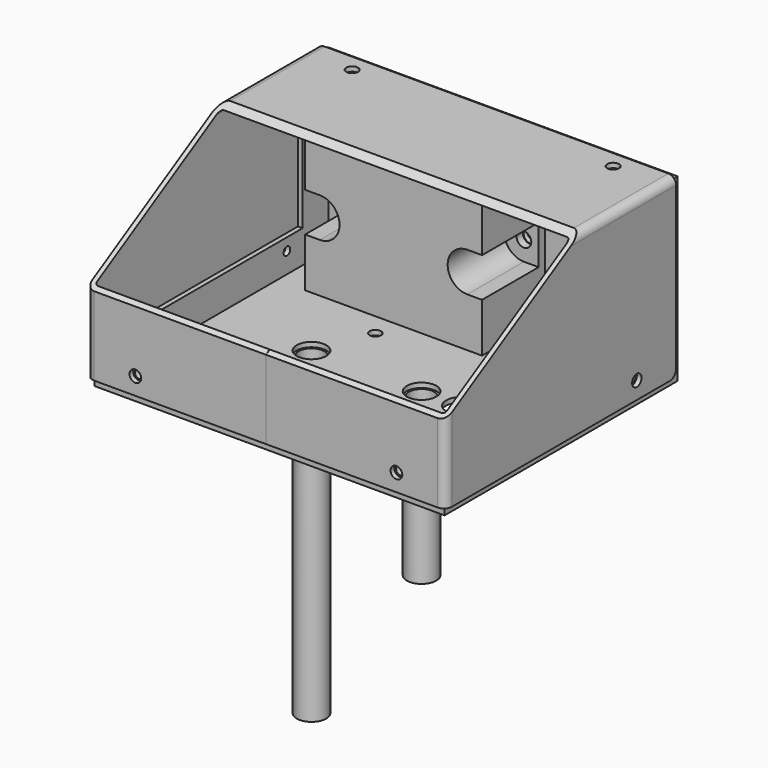
from build123d import *

# Parameters (mm, degrees)
F1_DEPTH         = 116.078
F2_R             = 2.54
F3_T             = -1.524
F5_DEPTH         = 113.03
F6_T             = -1.524
F7_W             = 57.15
F7_H             = 44.45
F8_DEPTH         = 25.4
F10_DEPTH        = 22.86
F11_R            = 2.3749
F12_DEPTH        = 26.925
F13_R            = 4.7625
F14_DEPTH        = 1.524
F15_R            = 4.7625
F15_R_2          = 4.1275
F16_DEPTH        = 50.8
F17_DEPTH        = 101.6
F18_R            = 1.8288
F19_DEPTH        = 59.691
F20_R            = 2.15265
F21_DEPTH        = 1.525
F22_R            = 9.525
F23_DEPTH        = 1.525
F27_D            = 3.7973
F27_ON_F25_D     = 3.7973
F27_ON_F24_D     = 3.7973
F28_D            = 2.7051
F29_D            = 2.7051
F29_DEPTH        = 12.7
F29_START        = 1.524
F29_TIP          = 0.8126940303
F29_ON_F25_D     = 2.7051
F29_ON_F25_DEPTH = 12.7
F29_ON_F25_START = 1.524
F29_ON_F25_TIP   = 0.8126940303
F30_W            = 0.0254
F30_H            = 69.686152041
F31_DEPTH        = 25.4
F32_R            = 2.54


with BuildPart() as f1:
    # F0 (on Right) → F1 (new body)
    with BuildSketch(Plane.YZ):
        Polygon((0, 25.4), (0, 0), (93.0926131403, 0), (93.0926131403, 57.15), (54.9926131403, 57.15), align=None)
    extrude(amount=F1_DEPTH)

    # F2
    f2_edges = [f1.edges().sort_by_distance(p)[0] for p in [
        (116.078, 74.042613, 57.15),
        (116.078, 0, 12.7),
        (0, 0, 12.7),
        (0, 74.042613, 57.15),
    ]]
    fillet(f2_edges, radius=F2_R)

    # F3
    f3_openings = [f1.faces().sort_by_distance(p)[0] for p in [
        (58.039, 93.092613, 28.563304),
        (58.039, 46.558092, 0),
        (58.039, 27.488057, 41.270237),
    ]]
    offset(amount=F3_T, openings=f3_openings)

    # F27 (through all)
    with Locations(Plane.XY.offset(57.15)):
        with Locations((100.203, 87.5046131403), (15.875, 87.5046131403)):
            Hole(F27_D / 2)

    # F27 on F25 (through all)
    with Locations(Plane.XZ):
        with Locations((15.875, 5.588), (100.203, 5.588)):
            Hole(F27_ON_F25_D / 2)

    # F27 on F24 (through all)
    with Locations(Plane(origin=(0, 0, 0), x_dir=(0, -1, 0), z_dir=(-1, 0, 0))):
        with Locations((-77.2176131403, 5.588)):
            Hole(F27_ON_F24_D / 2)

    # F30 (on face) → F31 (cut)
    with BuildSketch(Plane.XZ):
        with Locations((58.0517, 34.8430760205)):
            Rectangle(F30_W, F30_H)
    extrude(amount=-F31_DEPTH, mode=Mode.SUBTRACT)

    # F32
    f32_edges = [f1.edges().sort_by_distance(p)[0] for p in [
        (0.762, 93.092613, 0),
        (115.316, 93.092613, 0),
    ]]
    fillet(f32_edges, radius=F32_R)


with BuildPart() as f5:
    # F4 (on face) → F5 (new body, through all)
    with BuildSketch(Plane(origin=(114.554, 0, 0), x_dir=(0, -1, 0), z_dir=(-1, 0, 0))):
        Polygon((-1.524, 9.525), (-83.5676131403, 9.525), (-83.5676131403, 55.626), (-93.0926131403, 55.626), (-95.6326131403, 55.626), (-95.6326131403, -2.54), (-1.524, -2.54), (-1.524, 0), align=None)
    extrude(amount=F5_DEPTH)

    # F6
    f6_openings = [f5.faces().sort_by_distance(p)[0] for p in [
        (58.039, 83.567613, 32.5755),
        (58.039, 42.545807, 9.525),
    ]]
    offset(amount=F6_T, openings=f6_openings)

    # F13 (on face) → F14 (cut, through all)
    with BuildSketch(Plane(origin=(0, 0, -2.54), x_dir=(1, 0, 0), z_dir=(0, 0, -1))):
        with Locations((82.169, -48.5783125154)):
            Circle(F13_R)
        with Locations((69.469, -48.5783125154)):
            Circle(F13_R)
        with Locations((33.909, -48.5783125154)):
            Circle(F13_R)
    extrude(amount=-F14_DEPTH, mode=Mode.SUBTRACT)

    # F18 (on face) → F19 (cut, through all)
    with BuildSketch(Plane(origin=(0, 0, -2.54), x_dir=(1, 0, 0), z_dir=(0, 0, -1))):
        with Locations((40.5765, -31.1158125154)):
            Circle(F18_R)
        with Locations((75.5015, -31.1158125154)):
            Circle(F18_R)
        with Locations((75.5015, -66.0408125154)):
            Circle(F18_R)
        with Locations((40.5765, -66.0408125154)):
            Circle(F18_R)
    extrude(amount=-F19_DEPTH, mode=Mode.SUBTRACT)

    # F20 (on face) → F21 (cut, through all)
    with BuildSketch(Plane.XZ.offset(-94.1086131403)):
        with Locations((20.5105, 24.257)):
            Circle(F20_R)
        with Locations((68.1355, 24.257)):
            Circle(F20_R)
    extrude(amount=-F21_DEPTH, mode=Mode.SUBTRACT)

    # F22 (on face) → F23 (cut, through all)
    with BuildSketch(Plane.XZ.offset(-94.1086131403)):
        with Locations((92.964, 19.05)):
            Circle(F22_R)
    extrude(amount=-F23_DEPTH, mode=Mode.SUBTRACT)

    # F28 (through all)
    with Locations(Plane(origin=(0, 0, 0), x_dir=(0, -1, 0), z_dir=(-1, 0, 0))):
        with Locations((-77.2176131403, 5.588)):
            Hole(F28_D / 2)

    # F29
    # its depths count from where the whole tool has entered the part; down to there all is cleared
    with Locations(Plane.XY.offset(57.15).offset(-F29_START)):
        with Locations((15.875, 87.5046131403), (100.203, 87.5046131403)):
            Hole(F29_D / 2, depth=F29_DEPTH)
            with Locations((0, 0, -(F29_DEPTH + F29_TIP / 2))):  # 118° drill point
                Cone(0, F29_D / 2, F29_TIP, mode=Mode.SUBTRACT)

    # F29 on F25
    # its depths count from where the whole tool has entered the part; down to there all is cleared
    with Locations(Plane.XZ.offset(-F29_ON_F25_START)):
        with Locations((100.203, 5.588), (15.875, 5.588)):
            Hole(F29_ON_F25_D / 2, depth=F29_ON_F25_DEPTH)
            with Locations((0, 0, -(F29_ON_F25_DEPTH + F29_ON_F25_TIP / 2))):  # 118° drill point
                Cone(0, F29_ON_F25_D / 2, F29_ON_F25_TIP, mode=Mode.SUBTRACT)


with BuildPart() as f8:
    # F7 (on face) → F8 (new body)
    with BuildSketch(Plane.XZ.offset(-94.1086131403)):
        with Locations((44.323, 24.257)):
            Rectangle(F7_W, F7_H)
    extrude(amount=F8_DEPTH)

    # F9 (on face) → F10 (cut)
    with BuildSketch(Plane.XZ.offset(-68.7086131403)):
        with BuildLine():
            Line((72.898, 30.607), (68.1355, 30.607))
            ThreePointArc((68.1355, 30.607), (61.7855, 24.257), (68.1355, 17.907))
            Line((68.1355, 17.907), (72.898, 17.907))
            Line((72.898, 17.907), (72.898, 30.607))
        make_face()
        with BuildLine():
            ThreePointArc((20.5105, 17.907), (26.8605, 24.257), (20.5105, 30.607))
            Line((20.5105, 30.607), (15.748, 30.607))
            Line((15.748, 30.607), (15.748, 17.907))
            Line((15.748, 17.907), (20.5105, 17.907))
        make_face()
    extrude(amount=-F10_DEPTH, mode=Mode.SUBTRACT)

    # F11 (on face) → F12 (cut, through all)
    with BuildSketch(Plane.XZ.offset(-68.7086131403)):
        with BuildLine():
            Line((15.748, 21.8821), (20.5105, 21.8821))
            ThreePointArc((20.5105, 21.8821), (22.8854, 24.257), (20.5105, 26.6319))
            Line((20.5105, 26.6319), (15.748, 26.6319))
            Line((15.748, 26.6319), (15.748, 21.8821))
        make_face()
        with Locations((68.1355, 24.257)):
            Circle(F11_R)
    extrude(amount=-F12_DEPTH, mode=Mode.SUBTRACT)


with BuildPart() as f16:
    # F15 (on face) → F16 (new body)
    with BuildSketch(Plane(origin=(0, 0, -2.54), x_dir=(1, 0, 0), z_dir=(0, 0, -1))):
        with Locations((69.469, -48.5783125154)):
            Circle(F15_R)
        with Locations((69.469, -48.5783125154)):
            Circle(F15_R_2, mode=Mode.SUBTRACT)
    extrude(amount=F16_DEPTH)


with BuildPart() as f17:
    # F15 (on face) → F17 (new body)
    with BuildSketch(Plane(origin=(0, 0, -2.54), x_dir=(1, 0, 0), z_dir=(0, 0, -1))):
        with Locations((33.909, -48.5783125154)):
            Circle(F15_R)
        with Locations((33.909, -48.5783125154)):
            Circle(F15_R_2, mode=Mode.SUBTRACT)
    extrude(amount=F17_DEPTH)


solid = Compound([f1.part, f5.part, f8.part, f16.part, f17.part])
